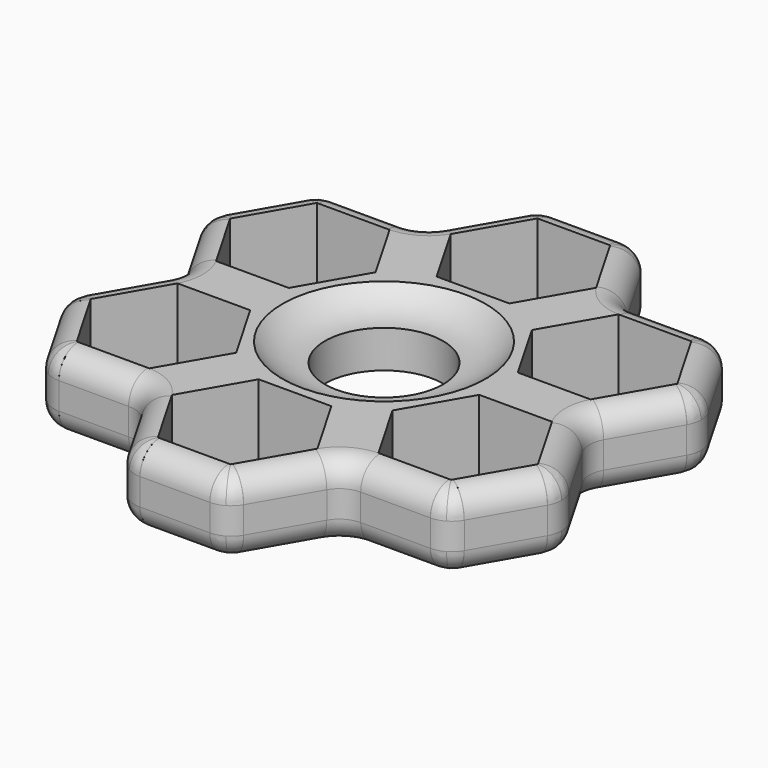
from build123d import *

# Parameters (mm, degrees)
F2_DEPTH = 7
F3_R     = 5
F4_R     = 4.49999
F1_R     = 11
F5_DEPTH = 12.5


# Not quite as in the source:
# - a fillet or chamfer is up to 0.001 mm smaller than in the source, because OpenCascade refuses the exact size


with BuildPart() as f2:
    # F0 (on Top) → F2 (new body, symmetric)
    with BuildSketch(Plane.XY):
        Polygon((-9.3819418743, 48.75), (-18.7638837487, 32.5), (-37.5277674973, 32.5), (-46.9097093717, 16.25), (-37.5277674973, 0), (-46.9097093717, -16.25), (-37.5277674973, -32.5), (-18.7638837487, -32.5), (-9.3819418743, -48.75), (9.3819418743, -48.75), (18.7638837487, -32.5), (37.5277674973, -32.5), (46.9097093717, -16.25), (37.5277674973, 0), (46.9097093717, 16.25), (37.5277674973, 32.5), (18.7638837487, 32.5), (9.3819418743, 48.75), align=None)
        Polygon((-13.567731326, -32.5), (-6.783865663, -20.75), (6.783865663, -20.75), (13.567731326, -32.5), (6.783865663, -44.25), (-6.783865663, -44.25), align=None, mode=Mode.SUBTRACT)
        Polygon((-21.36195996, -28), (-34.929691286, -28), (-41.713556949, -16.25), (-34.929691286, -4.5), (-21.36195996, -4.5), (-14.578094297, -16.25), align=None, mode=Mode.SUBTRACT)
        Polygon((41.713556949, -16.25), (34.929691286, -28), (21.36195996, -28), (14.578094297, -16.25), (21.36195996, -4.5), (34.929691286, -4.5), align=None, mode=Mode.SUBTRACT)
        Polygon((-34.929691286, 4.5), (-41.713556949, 16.25), (-34.929691286, 28), (-21.36195996, 28), (-14.578094297, 16.25), (-21.36195996, 4.5), align=None, mode=Mode.SUBTRACT)
        Polygon((-6.783865663, 44.25), (6.783865663, 44.25), (13.567731326, 32.5), (6.783865663, 20.75), (-6.783865663, 20.75), (-13.567731326, 32.5), align=None, mode=Mode.SUBTRACT)
        Polygon((34.929691286, 28), (41.7135569489, 16.25), (34.929691286, 4.5), (21.36195996, 4.5), (14.578094297, 16.25), (21.36195996, 28), align=None, mode=Mode.SUBTRACT)
    extrude(amount=F2_DEPTH, both=True)

    # F3
    f3_edges = [f2.edges().sort_by_distance(p)[0] for p in [
        (18.763884, -32.5, 0),
        (9.381942, -48.75, 0),
        (-9.381942, -48.75, 0),
        (-37.527767, -32.5, 0),
        (37.527767, -32.5, 0),
        (46.909709, -16.25, 0),
        (46.909709, 16.25, 0),
        (-18.763884, -32.5, 0),
        (-46.909709, -16.25, 0),
        (-37.527767, 0, 0),
        (-46.909709, 16.25, 0),
        (-37.527767, 32.5, 0),
        (-18.763884, 32.5, 0),
        (-9.381942, 48.75, 0),
        (9.381942, 48.75, 0),
        (18.763884, 32.5, 0),
        (37.527767, 32.5, 0),
        (37.527767, 0, 0),
    ]]
    fillet(f3_edges, radius=F3_R)

    # F4 (radius 4.5 in the source; OpenCascade refuses exactly that, so slightly less here)
    f4_edges = [f2.edges().sort_by_distance(p)[0] for p in [
        (-42.218738, -24.375, 7),
        (-42.218738, -24.375, -7),
    ]]
    fillet(f4_edges, radius=F4_R)

    # F1 (on Top) → F5 (cut, symmetric)
    with BuildSketch(Plane.XY):
        Circle(F1_R)
    extrude(amount=F5_DEPTH, both=True, mode=Mode.SUBTRACT)

    # F6 (on Right) → F7 (revolve, cut)
    with BuildSketch(Plane.YZ):
        with BuildLine():
            Line((-11, 7), (-18.95, 7))
            ThreePointArc((-18.95, 7), (-15.3431699253, 4.4137283125), (-11, 3.5))
            Line((-11, 3.5), (-11, 7))
        make_face()
        with BuildLine():
            Line((-11, -7), (-11, -3.5))
            ThreePointArc((-11, -3.5), (-15.3431699253, -4.4137283125), (-18.95, -7))
            Line((-18.95, -7), (-11, -7))
        make_face()
    revolve(axis=Axis((0, 0, 7.0033883676), (0, 0, 1)), mode=Mode.SUBTRACT)


solid = f2.part
